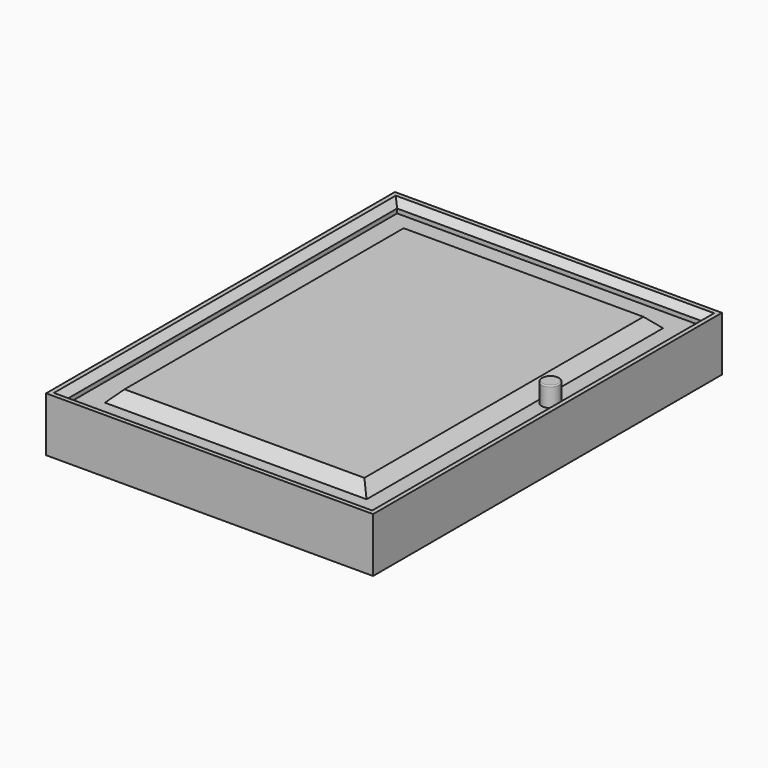
from build123d import *

# Parameters (mm, degrees)
F0_W     = 1500
F0_H     = 2000
F0_W_2   = 1400
F0_H_2   = 1900
F0_W_3   = 1200
F0_H_3   = 1700
F1_DEPTH = 125
F2_W     = 1400
F2_H     = 1900
F2_W_2   = 1200
F2_H_2   = 1700
F3_DEPTH = 50
F4_SIZE  = 49.99999
F5_SIZE  = 30
F6_R     = 40
F7_DEPTH = 90
F8_R     = 5


# Not quite as in the source:
# - a fillet or chamfer is up to 0.001 mm smaller than in the source, because OpenCascade refuses the exact size


with BuildPart() as f1:
    # F0 (on Top) → F1 (new body, symmetric)
    with BuildSketch(Plane.XY):
        Rectangle(F0_W, F0_H)
        Rectangle(F0_W_2, F0_H_2, mode=Mode.SUBTRACT)
        Rectangle(F0_W_2, F0_H_2)
        Rectangle(F0_W_3, F0_H_3, mode=Mode.SUBTRACT)
        Rectangle(F0_W_3, F0_H_3)
    extrude(amount=F1_DEPTH, both=True)

    # F2 (on face) → F3 (cut)
    with BuildSketch(Plane.XY.offset(125)):
        Rectangle(F2_W, F2_H)
        Rectangle(F2_W_2, F2_H_2, mode=Mode.SUBTRACT)
    extrude(amount=-F3_DEPTH, mode=Mode.SUBTRACT)

    # F4 (size 50 in the source; OpenCascade refuses exactly that, so slightly less here)
    f4_edges = [f1.edges().sort_by_distance(p)[0] for p in [
        (-600, 0, 125),
        (0, 850, 125),
        (600, 0, 125),
        (0, -850, 125),
    ]]
    chamfer(f4_edges, length=F4_SIZE)

    # F5
    f5_edges = [f1.edges().sort_by_distance(p)[0] for p in [
        (-700, 0, 125),
        (0, 950, 125),
        (700, 0, 125),
        (0, -950, 125),
    ]]
    chamfer(f5_edges, length=F5_SIZE)

    # F6 (on face) → F7 (join)
    with BuildSketch(Plane.XY.offset(75)):
        with Locations((647.2854614258, 145.2714502811)):
            Circle(F6_R)
    extrude(amount=F7_DEPTH)

    # F8
    f8_edges = [f1.edges().sort_by_distance(p)[0] for p in [
        (607.285461, 145.27145, 165),
    ]]
    fillet(f8_edges, radius=F8_R)


solid = f1.part
